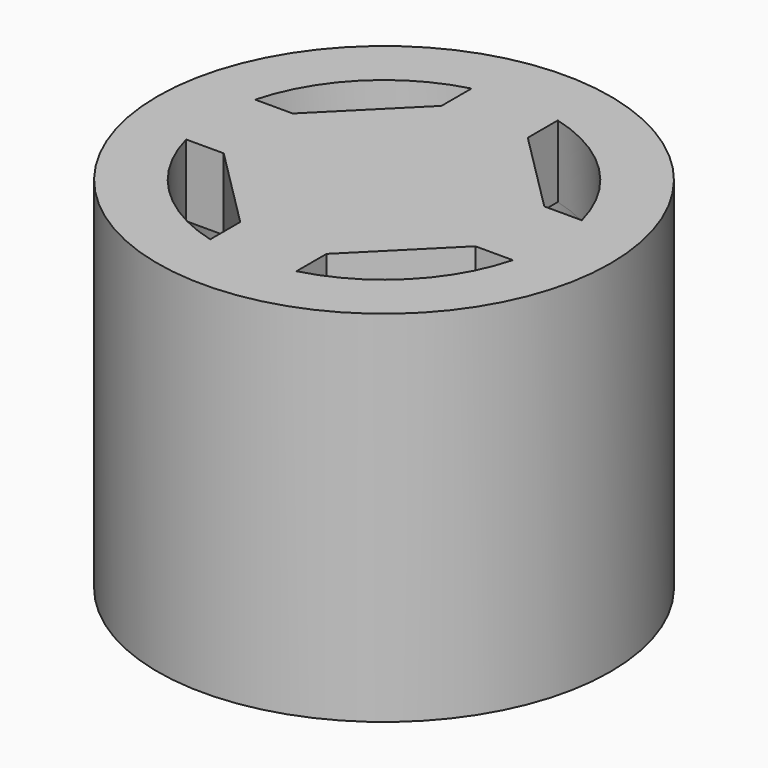
from build123d import *

# Parameters (mm, degrees)
F0_R     = 3.15
F0_R_2   = 2.35
F1_DEPTH = 4
F2_R     = 3.15
F3_DEPTH = 1


# Not quite as in the source:
# - after a boolean that leaves OpenCascade's solid faulty, fix() repairs it


with BuildPart() as f1:
    # F0 (on Top) → F1 (new body)
    with BuildSketch(Plane.XY):
        Circle(F0_R)
        Circle(F0_R_2, mode=Mode.SUBTRACT)
    extrude(amount=F1_DEPTH)

    # F2 (on face) → F3 (join)
    with BuildSketch(Plane.XY.offset(4)):
        Circle(F2_R)
        with BuildLine():
            ThreePointArc((-2.2721135535, 0.6), (-1.6617009358, 1.6617009358), (-0.6, 2.2721135535))
            ThreePointArc((-0.6, 2.2721135535), (0, 2.35), (0.6, 2.2721135535))
            ThreePointArc((0.6, 2.2721135535), (1.6617009358, 1.6617009358), (2.2721135535, 0.6))
            ThreePointArc((2.2721135535, 0.6), (2.3304470441, 0.302517065), (2.35, 0))
            ThreePointArc((2.35, 0), (2.3304470441, -0.302517065), (2.2721135535, -0.6))
            ThreePointArc((2.2721135535, -0.6), (1.6617009358, -1.6617009358), (0.6, -2.2721135535))
            ThreePointArc((0.6, -2.2721135535), (0, -2.35), (-0.6, -2.2721135535))
            ThreePointArc((-0.6, -2.2721135535), (-1.6617009358, -1.6617009358), (-2.2721135535, -0.6))
            ThreePointArc((-2.2721135535, -0.6), (-2.35, 0), (-2.2721135535, 0.6))
        make_face(mode=Mode.SUBTRACT)
        with BuildLine():
            ThreePointArc((0.6, 2.2721135535), (0, 2.35), (-0.6, 2.2721135535))
            Line((-0.6, 2.2721135535), (-0.6, 1.75))
            Line((-0.6, 1.75), (-1.75, 0.6))
            Line((-1.75, 0.6), (-2.2721135535, 0.6))
            ThreePointArc((-2.2721135535, 0.6), (-2.35, 0), (-2.2721135535, -0.6))
            Line((-2.2721135535, -0.6), (-1.75, -0.6))
            Line((-1.75, -0.6), (-0.6, -1.75))
            Line((-0.6, -1.75), (-0.6, -2.2721135535))
            ThreePointArc((-0.6, -2.2721135535), (0, -2.35), (0.6, -2.2721135535))
            Line((0.6, -2.2721135535), (0.6, -1.75))
            Line((0.6, -1.75), (1.75, -0.6))
            Line((1.75, -0.6), (2.2721135535, -0.6))
            ThreePointArc((2.2721135535, -0.6), (2.3304470441, -0.302517065), (2.35, 0))
            ThreePointArc((2.35, 0), (2.3304470441, 0.302517065), (2.2721135535, 0.6))
            Line((2.2721135535, 0.6), (1.75, 0.6))
            Line((1.75, 0.6), (0.6, 1.75))
            Line((0.6, 1.75), (0.6, 2.2721135535))
        make_face()
    extrude(amount=F3_DEPTH)

    add(f1.part.fix(), mode=Mode.REPLACE)


solid = f1.part
